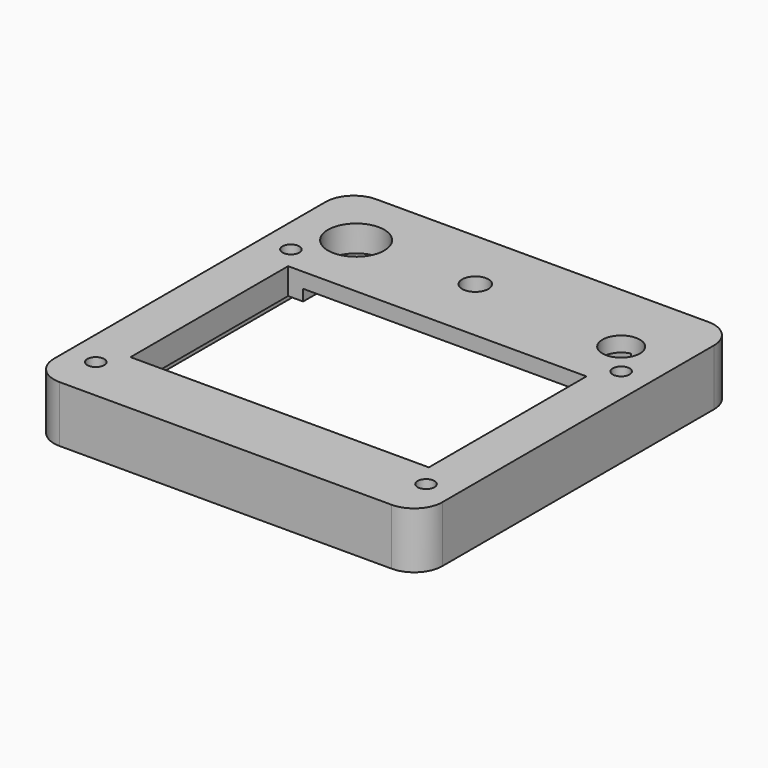
from build123d import *

# Parameters (mm, degrees)
F0_R     = 2.25
F0_W     = 79.5
F0_H     = 52.5
F1_DEPTH = 15
F2_W     = 8.5
F2_H     = 42.5
F2_W_2   = 71.5
F2_H_2   = 25
F3_DEPTH = 11
F4_W     = 96
F4_H     = 90
F5_DEPTH = 8
F6_R     = 7.5
F6_R_2   = 3.5
F6_R_3   = 5
F7_DEPTH = 15.001
F8_R     = 7.5


with BuildPart() as f1:
    # F0 (on Top) → F1 (new body)
    with BuildSketch(Plane.XY):
        Polygon((-51.75, -9.25), (-51.75, -44.25), (51.75, -44.25), (51.75, 61.25), (11.75, 61.25), (-3.25, 61.25), (-51.75, 61.25), align=None)
        with Locations((-44, -32.5)):
            Circle(F0_R, mode=Mode.SUBTRACT)
        with Locations((44, -32.5)):
            Circle(F0_R, mode=Mode.SUBTRACT)
        Rectangle(F0_W, F0_H, mode=Mode.SUBTRACT)
        with Locations((-44, 32.5)):
            Circle(F0_R, mode=Mode.SUBTRACT)
        with Locations((44, 32.5)):
            Circle(F0_R, mode=Mode.SUBTRACT)
    extrude(amount=F1_DEPTH)

    # F2 (on face) → F3 (cut)
    with BuildSketch(Plane(origin=(0, 0, 0), x_dir=(1, 0, 0), z_dir=(0, 0, -1))):
        with Locations((44, 0)):
            Rectangle(F2_W, F2_H)
        with Locations((0, -38.75)):
            Rectangle(F2_W_2, F2_H_2)
    extrude(amount=-F3_DEPTH, mode=Mode.SUBTRACT)

    # F4 (on face) → F5 (cut)
    with BuildSketch(Plane(origin=(0, 0, 0), x_dir=(1, 0, 0), z_dir=(0, 0, -1))):
        with Locations((-0.25, -8.25)):
            Rectangle(F4_W, F4_H)
    extrude(amount=-F5_DEPTH, mode=Mode.SUBTRACT)

    # F6 (on face) → F7 (cut, through all)
    with BuildSketch(Plane.XY.offset(15)):
        with Locations((-36.025, 44.25)):
            Circle(F6_R)
        with Locations((-4.275, 44.25)):
            Circle(F6_R_2)
        with Locations((37, 41.25)):
            Circle(F6_R_3)
    extrude(amount=-F7_DEPTH, mode=Mode.SUBTRACT)

    # F8
    f8_edges = [f1.edges().sort_by_distance(p)[0] for p in [
        (51.75, -44.25, 7.5),
        (-51.75, 61.25, 7.5),
        (-51.75, -44.25, 7.5),
        (51.75, 61.25, 7.5),
    ]]
    fillet(f8_edges, radius=F8_R)


solid = f1.part
